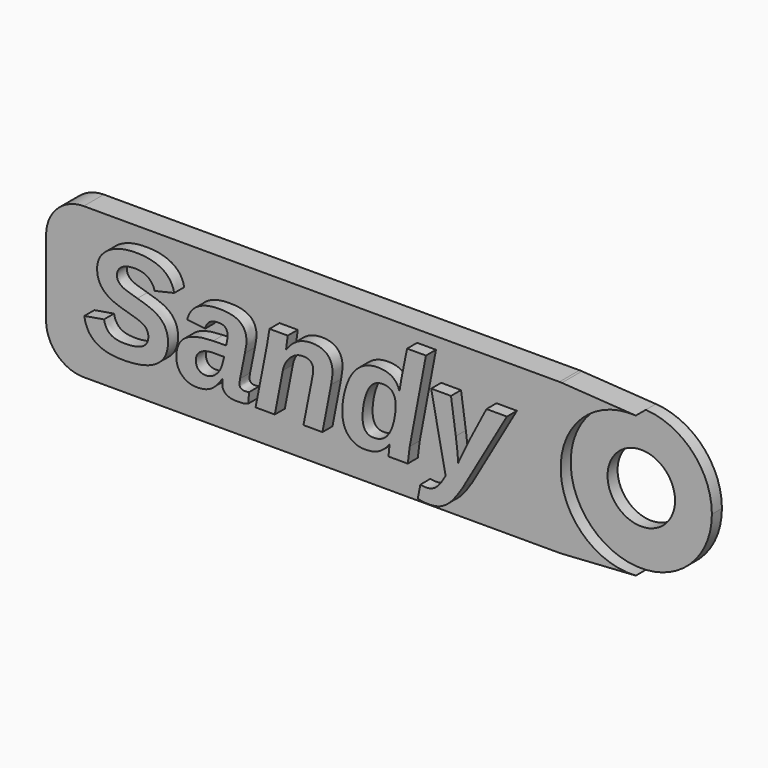
from build123d import *

# Parameters (mm, degrees)
F0_TEXT_SIZE = 11.1111111111
F1_DEPTH     = 1
F2_R         = 2.69
F3_DEPTH     = 2
F4_T1_DEPTH  = 17
F4_T3_DEPTH  = 2.4838709677
F5_R         = 5.625
F6_DEPTH     = 1


# Not quite as in the source:
# - a fillet or chamfer that OpenCascade refuses, or shapes differently, is made with other operations: its cross-section is extruded or revolved along the edge and cut away or added
# - Text() gives the source's letters only with a copy of the font that has no kerning and outlines rounded to 1/6400 em; it was checked with that copy


with BuildPart() as f1:
    # F0 (on Front) → F1 (new body)
    with BuildSketch(Plane.XZ):
        with Locations((-17.2873263889, -8)):
            Text('Sandy', F0_TEXT_SIZE, font='Arimo', font_style=FontStyle.BOLDITALIC, text_align=(TextAlign.LEFT, TextAlign.BOTTOM))
    extrude(amount=F1_DEPTH)


with BuildPart() as f3:
    # F2 (on Front) → F3 (new body)
    with BuildSketch(Plane.XZ):
        with BuildLine():
            Line((-21, -11), (20, -11))
            Line((20, -11), (25.9875259875, -10.6133056133))
            ThreePointArc((25.9875259875, -10.6133056133), (20, -5), (25.9875259875, 0.6133056133))
            Line((25.9875259875, 0.6133056133), (20, 1))
            Line((20, 1), (-21, 1))
            Line((-21, 1), (-21, -11))
        make_face()
        with BuildLine():
            ThreePointArc((25.9875259875, 0.6133056133), (20, -5), (25.9875259875, -10.6133056133))
            ThreePointArc((25.9875259875, -10.6133056133), (29.7286467733, -8.84716885), (31.25, -5))
            ThreePointArc((31.25, -5), (29.7286467733, -1.15283115), (25.9875259875, 0.6133056133))
        make_face()
        with Locations((25.625, -5)):
            Circle(F2_R, mode=Mode.SUBTRACT)
    extrude(amount=-F3_DEPTH)

    # F4: fillet of radius 3 on 4 edges, made by hand

    # F4_s2 → F4_t1 (cut)
    with BuildSketch(Plane.XZ.offset(-9.5)):
        with BuildLine():
            ThreePointArc((-18, 1), (-20.1213203436, 0.1213203436), (-21, -2))
            Line((-21, -2), (-21, 1))
            Line((-21, 1), (-18, 1))
        make_face()
        with BuildLine():
            ThreePointArc((-18, -11), (-20.1213203436, -10.1213203436), (-21, -8))
            Line((-21, -8), (-21, -11))
            Line((-21, -11), (-18, -11))
        make_face()
    extrude(amount=F4_T1_DEPTH, mode=Mode.SUBTRACT)

    # F4_s4 → F4_t3 (cut)
    with BuildSketch(Plane.XZ.offset(-2.2419354839)):
        with BuildLine():
            ThreePointArc((19.9032258065, -11), (19.9999496885, -10.998440343), (20.0965729998, -10.9937629938))
            Line((20.0965729998, -10.9937629938), (20, -11))
            Line((20, -11), (19.9032258065, -11))
        make_face()
        with BuildLine():
            ThreePointArc((20.0965729998, 0.9937629938), (19.9999496885, 0.998440343), (19.9032258065, 1))
            Line((19.9032258065, 1), (20, 1))
            Line((20, 1), (20.0965729998, 0.9937629938))
        make_face()
    extrude(amount=F4_T3_DEPTH, mode=Mode.SUBTRACT)

    # F5 (on face) → F6 (cut)
    with BuildSketch(Plane.XZ):
        with Locations((25.625, -5)):
            Circle(F5_R)
    extrude(amount=-F6_DEPTH, mode=Mode.SUBTRACT)


solid = Compound([f1.part, f3.part])
